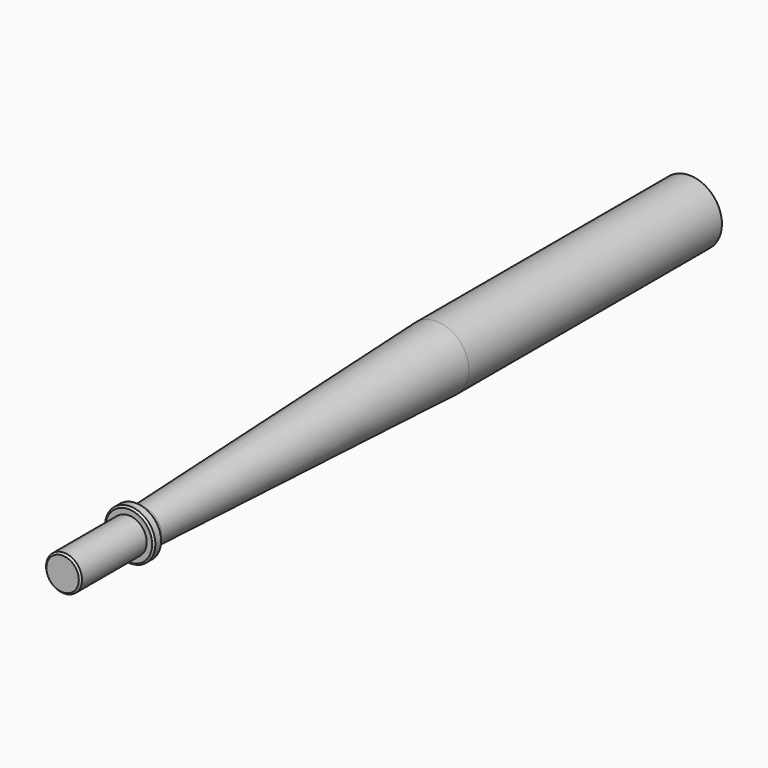
from build123d import *

# Parameters (mm, degrees)
F2_SIZE = 0.5


# Not quite as in the source:
# - a fillet or chamfer that OpenCascade refuses, or shapes differently, is made with other operations: its cross-section is extruded or revolved along the edge and cut away or added


with BuildPart() as f1:
    # F0 (on Right) → F1 (revolve)
    with BuildSketch(Plane.YZ):
        Polygon((103.6051637142, 6), (103.6051637142, 9), (15.6051637142, 9), (-88.3948362864, 5), (-88.3948362864, 7), (-91.3948362864, 7), (-91.3948362864, 5), (-114.3948362864, 5), (-114.3948362864, 0), (0, 0), (3.6051637142, 6), align=None)
    revolve(axis=Axis((0, -57.1974181432, 0), (0, -1, 0)))

    # F2
    f2_edges = [f1.edges().sort_by_distance(p)[0] for p in [
        (0, -91.394836, -7),
        (0, -88.394836, -7),
        (0, -114.394836, -5),
    ]]
    chamfer(f2_edges, length=F2_SIZE)

    # F3: fillet of radius 2 on 1 edges, made by hand

    # F3_s1 → F3_t2 (revolve)
    with BuildSketch(Plane.YZ):
        with BuildLine():
            ThreePointArc((-88.3948362864, 6.5), (-87.641927013, 5.4477782371), (-86.4024545248, 5.0766300678))
            Line((-86.4024545248, 5.0766300678), (-86.4009172, 5.0366596208))
            Line((-86.4009172, 5.0366596208), (-88.3932989615, 4.960029553))
            Line((-88.3932989615, 4.960029553), (-88.4348362864, 5))
            ThreePointArc((-88.4348362864, 5), (-88.4348362864, 5.75), (-88.4331465967, 6.4884969517))
            Line((-88.4331465967, 6.4884969517), (-88.3948362864, 6.5))
        make_face()
    revolve(axis=Axis((0, -88.3948362864, 0), (0, -1, 0)))


solid = f1.part
